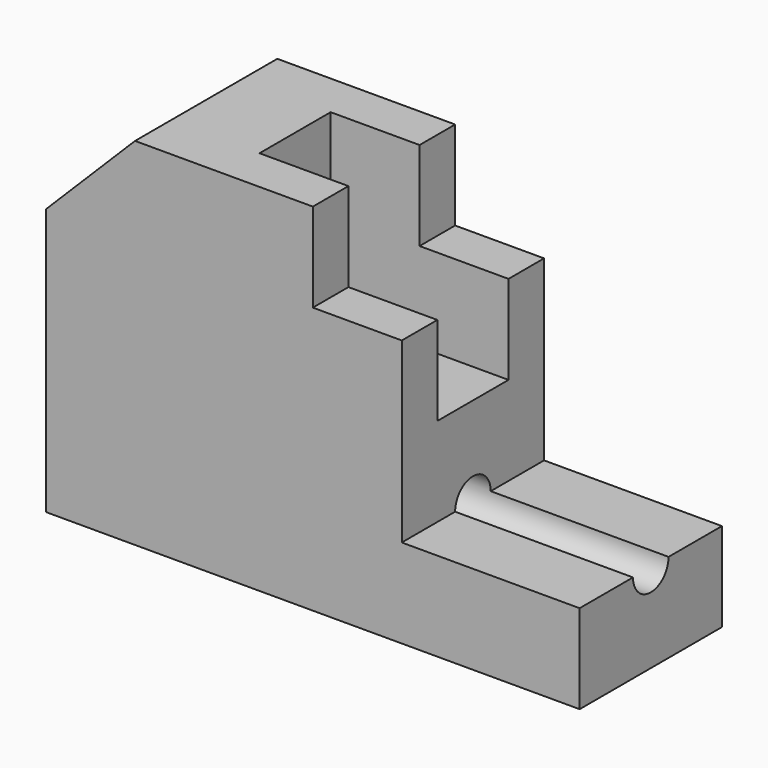
from build123d import *

# Parameters (mm, degrees)
F1_DEPTH = 12.7
F4_DEPTH = 6.35
F5_R     = 3.175
F6_DEPTH = 76.201


# Not quite as in the source:
# - a feature of the source that left no trace in its solid (it failed there, or was rolled back) is left out


with BuildPart() as f1:
    # F0 (on Front) → F1 (new body, symmetric)
    with BuildSketch(Plane.XZ):
        Polygon((0, 38.1), (0, 0), (76.2, 0), (76.2, 12.7), (50.8, 12.7), (50.8, 38.1), (38.1, 38.1), (38.1, 50.8), (12.7, 50.8), align=None)
    extrude(amount=F1_DEPTH, both=True)

    # F2 (on Front) → F4 (cut, symmetric)
    with BuildSketch(Plane.XZ):
        Polygon((38.1, 50.8), (25.4, 50.8), (25.4, 25.4), (50.8, 25.4), (50.8, 38.1), (38.1, 38.1), align=None)
    extrude(amount=F4_DEPTH, both=True, mode=Mode.SUBTRACT)

    # F5 (on Right) → F6 (cut, through all)
    with BuildSketch(Plane.YZ):
        with Locations((0, 12.7)):
            Circle(F5_R)
    extrude(amount=F6_DEPTH, mode=Mode.SUBTRACT)


solid = f1.part
